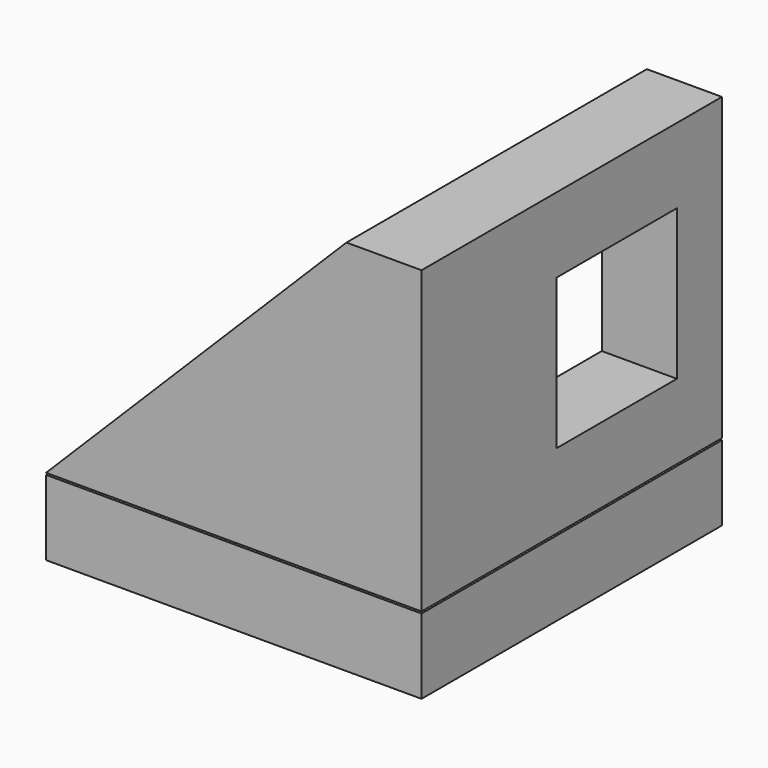
from build123d import *

# Parameters (mm, degrees)
F0_W      = 100
F0_H      = 100
F1_DEPTH  = 20
F2_W      = 100
F2_H      = 80
F3_DEPTH  = 20
F4_R      = 15
F5_DEPTH  = 21
F6_W      = 80
F6_H      = 80
F7_DEPTH  = 30
F8_SIZE   = 79.99999
F9_W      = 40
F9_H      = 40
F10_DEPTH = 22
F11_R     = 20


# Not quite as in the source:
# - a fillet or chamfer is up to 0.001 mm smaller than in the source, because OpenCascade refuses the exact size


with BuildPart() as f1:
    # F0 (on Top) → F1 (new body)
    with BuildSketch(Plane.XY):
        with Locations((-50, -50)):
            Rectangle(F0_W, F0_H)
    extrude(amount=F1_DEPTH)

    # F4 (on face) → F5 (cut)
    with BuildSketch(Plane.XY.offset(20)):
        with Locations((-75, -25)):
            Circle(F4_R)
    extrude(amount=-F5_DEPTH, mode=Mode.SUBTRACT)

    # F11
    f11_edges = [f1.edges().sort_by_distance(p)[0] for p in [
        (-100, 0, 10),
    ]]
    fillet(f11_edges, radius=F11_R)


with BuildPart() as f3:
    # F2 (on Right) → F3 (new body)
    with BuildSketch(Plane.YZ):
        with Locations((-50, 60.4958688773)):
            Rectangle(F2_W, F2_H)
    extrude(amount=-F3_DEPTH)

    # F6 (on face) → F7 (join)
    with BuildSketch(Plane.XZ.offset(100)):
        with Locations((-60, 60.4958688773)):
            Rectangle(F6_W, F6_H)
    extrude(amount=-F7_DEPTH)

    # F8 (size 80 in the source; OpenCascade refuses exactly that, so slightly less here)
    f8_edges = [f3.edges().sort_by_distance(p)[0] for p in [
        (-100, -85, 100.495869),
    ]]
    chamfer(f8_edges, length=F8_SIZE)

    # F9 (on face) → F10 (cut)
    with BuildSketch(Plane(origin=(-20, 0, 0), x_dir=(0, -1, 0), z_dir=(-1, 0, 0))):
        with Locations((35, 60.4958688773)):
            Rectangle(F9_W, F9_H)
    extrude(amount=-F10_DEPTH, mode=Mode.SUBTRACT)


solid = Compound([f1.part, f3.part])
